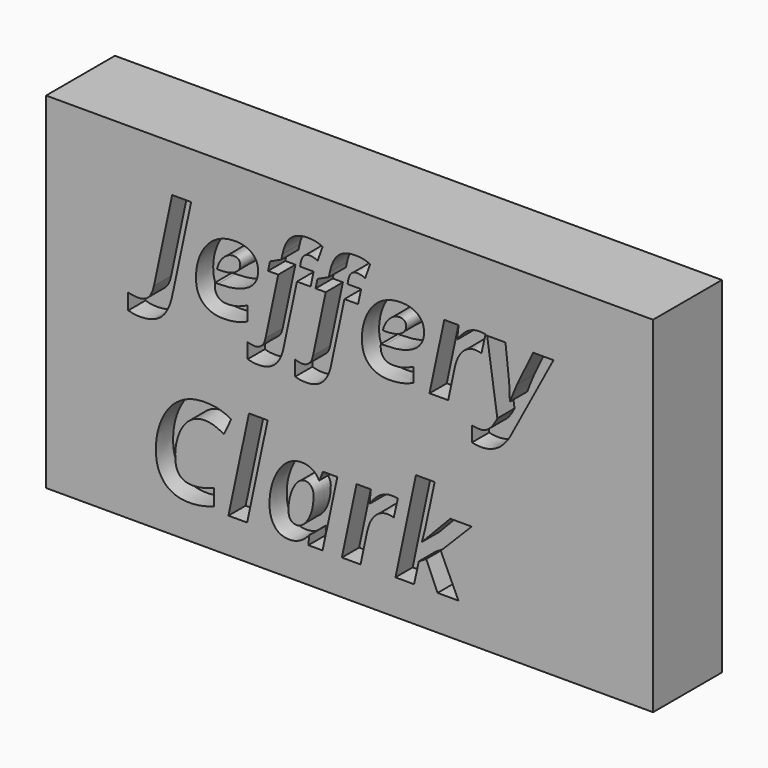
from build123d import *

# Parameters (mm, degrees)
F1_DEPTH     = 25.4
F2_TEXT_SIZE = 37.554711
F3_DEPTH     = 6.35
F4_TEXT_SIZE = 35.0921062313
F5_DEPTH     = 6.35


# Not quite as in the source:
# - Text() gives the source's letters only with a copy of the font that has no kerning and outlines rounded to 1/6400 em; it was checked with that copy


with BuildPart() as f1:
    # F0 (on Front) → F1 (new body)
    with BuildSketch(Plane.XZ):
        Polygon((-18.6172854155, 41.8888889253), (-67.3768445849, 41.8888889253), (-67.3768445849, -60.0629113615), (111.7037087679, -60.0629113615), (111.7037087679, 41.8888889253), (-3.5461494699, 41.8888889253), align=None)
    extrude(amount=F1_DEPTH)

    # F2 (on face) → F3 (cut)
    with BuildSketch(Plane.XZ.offset(25.4)):
        with Locations((-37.2345717624, 1.3298038393)):
            Text('Jeffery', F2_TEXT_SIZE, font='Open Sans', font_style=FontStyle.BOLDITALIC, text_align=(TextAlign.LEFT, TextAlign.BOTTOM))
        with Locations((-37.2345717624, -49.7446031206)):
            Text('Clark', F2_TEXT_SIZE, font='Open Sans', font_style=FontStyle.BOLDITALIC, text_align=(TextAlign.LEFT, TextAlign.BOTTOM))
    extrude(amount=-F3_DEPTH, mode=Mode.SUBTRACT)

    # F4 (on face) → F5 (cut)
    with BuildSketch(Plane(origin=(0, 0, 0), x_dir=(-1, 0, 0), z_dir=(0, 1, 0))):
        with Locations((-76.0627947748, 2.6596123353)):
            Text('Jeffery', F4_TEXT_SIZE, font='Open Sans', font_style=FontStyle.BOLDITALIC, text_align=(TextAlign.LEFT, TextAlign.BOTTOM))
        with Locations((-76.0627947748, -45.0656521393)):
            Text('Clark', F4_TEXT_SIZE, font='Open Sans', font_style=FontStyle.BOLDITALIC, text_align=(TextAlign.LEFT, TextAlign.BOTTOM))
    extrude(amount=-F5_DEPTH, mode=Mode.SUBTRACT)


solid = f1.part
